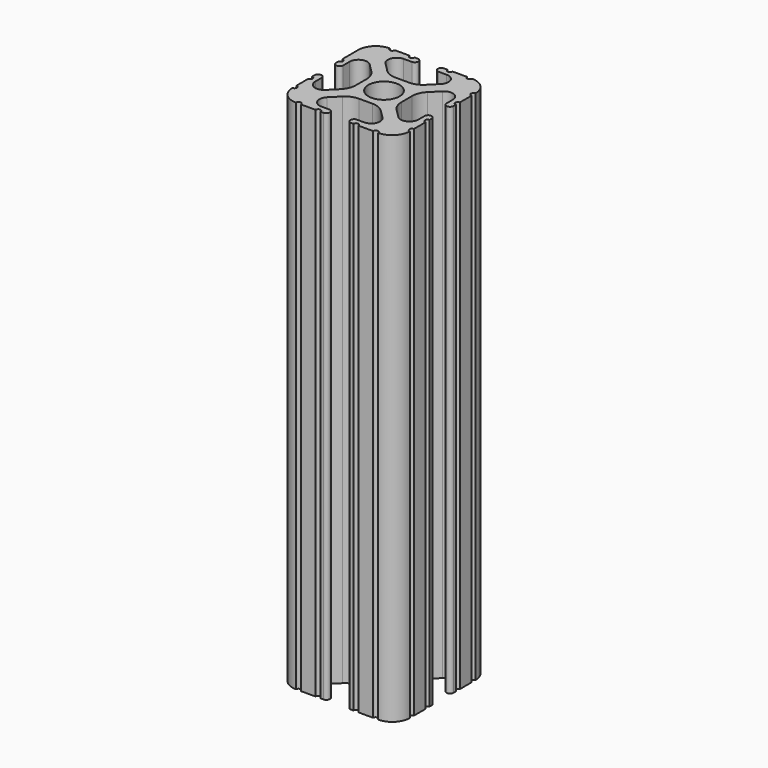
from build123d import *

# Parameters (mm, degrees)
F0_R     = 3.3625011168
F1_DEPTH = 111.76


# Not quite as in the source:
# - ends of sketch curves that miss each other by under 0.0002 mm in the source are joined


with BuildPart() as f1:
    # F0 (on Top) → F1 (new body)
    with BuildSketch(Plane.XY):
        with BuildLine():
            ThreePointArc((3.5659002011, 5.7489795053), (2.3298472421, 4.9230753228), (0.8718233648, 4.6330563417))
            Line((0.8718233648, 4.6330563417), (-2.0428700475, 4.6330563417))
            ThreePointArc((-2.0428700475, 4.6330563417), (-3.5008939248, 4.9230753228), (-4.7369468838, 5.7489795053))
            Line((-4.7369468838, 5.7489795053), (-6.5824285393, 7.5944611609))
            ThreePointArc((-6.5824285393, 7.5944611609), (-6.9953806306, 9.6705115177), (-5.2353901211, 10.846499579))
            Line((-5.2353901211, 10.846499579), (-3.5008939248, 10.846499579))
            Line((-3.5008939248, 10.846499579), (-3.4685428807, 10.846499579))
            ThreePointArc((-3.4685428807, 10.846499579), (-2.7109282724, 11.6201206221), (-3.4685428807, 12.3937416652))
            Line((-3.4685428807, 12.3937416652), (-3.5008939248, 12.3937416652))
            Line((-3.5008939248, 12.3937416652), (-4.1388643307, 12.3937416652))
            ThreePointArc((-4.1388643307, 12.3937416652), (-4.6871272259, 11.8525139305), (-5.2353901211, 12.3937416652))
            Line((-5.2353901211, 12.3937416652), (-8.3730050695, 12.3937416652))
            ThreePointArc((-8.3730050695, 12.3937416652), (-8.9242642054, 11.8424825293), (-9.4755233413, 12.3937416652))
            ThreePointArc((-9.4755233413, 12.3937416652), (-12.1696001777, 11.2778185015), (-13.2855233413, 8.5837416652))
            Line((-13.2855233413, 8.5837416652), (-13.2855233413, 7.4984658996))
            Line((-13.2855233413, 7.4984658996), (-13.2855233413, 4.343608445))
            ThreePointArc((-13.2855233413, 4.343608445), (-12.7296839168, 3.7964165708), (-13.2855233413, 3.2492246965))
            Line((-13.2855233413, 3.2492246965), (-13.2855233413, 2.6091122487))
            ThreePointArc((-13.2855233413, 2.6091122487), (-12.5119022982, 1.8532957784), (-11.7382812551, 2.6091122487))
            Line((-11.7382812551, 2.6091122487), (-11.7382812551, 4.343608445))
            ThreePointArc((-11.7382812551, 4.343608445), (-10.5622931938, 6.1035989545), (-8.486242837, 5.6906468632))
            Line((-8.486242837, 5.6906468632), (-6.6407611815, 3.8451652077))
            ThreePointArc((-6.6407611815, 3.8451652077), (-5.8148569989, 2.6091122487), (-5.5248380178, 1.1510883714))
            Line((-5.5248380178, 1.1510883714), (-5.5248380178, -1.7636050409))
            ThreePointArc((-5.5248380178, -1.7636050409), (-5.8148569989, -3.2216289182), (-6.6407611815, -4.4576818772))
            Line((-6.6407611815, -4.4576818772), (-8.486242837, -6.3031635328))
            ThreePointArc((-8.486242837, -6.3031635328), (-10.5622931938, -6.716115624), (-11.7382812551, -4.9561251146))
            Line((-11.7382812551, -4.9561251146), (-11.7382812551, -3.2216289182))
            ThreePointArc((-11.7382812551, -3.2216289182), (-12.5119022982, -2.4480078751), (-13.2855233413, -3.2216289182))
            Line((-13.2855233413, -3.2216289182), (-13.2855233413, -3.8570189362))
            Line((-13.2855233413, -3.8570189362), (-13.2855233413, -3.8595993241))
            ThreePointArc((-13.2855233413, -3.8595993241), (-12.7442956066, -4.4078622194), (-13.2855233413, -4.9561251146))
            Line((-13.2855233413, -4.9561251146), (-13.2855233413, -8.093740063))
            ThreePointArc((-13.2855233413, -8.093740063), (-12.9963771793, -8.175658031), (-12.7931661592, -8.3970656592))
            ThreePointArc((-12.7931661592, -8.3970656592), (-12.8130701183, -8.9360625991), (-13.2855233413, -9.1962583348))
            ThreePointArc((-13.2855233413, -9.1962583348), (-12.1696001777, -11.8903351711), (-9.4755233413, -13.0062583348))
            ThreePointArc((-9.4755233413, -13.0062583348), (-8.9263401234, -12.4513735034), (-8.3771569056, -13.0062583348))
            Line((-8.3771569056, -13.0062583348), (-5.2353901211, -13.0062583348))
            ThreePointArc((-5.2353901211, -13.0062583348), (-4.6881982469, -12.4504189103), (-4.1410063726, -13.0062583348))
            Line((-4.1410063726, -13.0062583348), (-3.5008939248, -13.0062583348))
            ThreePointArc((-3.5008939248, -13.0062583348), (-2.7450774545, -12.2326372917), (-3.5008939248, -11.4590162486))
            Line((-3.5008939248, -11.4590162486), (-5.2353901211, -11.4590162486))
            ThreePointArc((-5.2353901211, -11.4590162486), (-6.9953806306, -10.2830281872), (-6.5824285393, -8.2069778304))
            ThreePointArc((-6.5824285393, -8.2069778304), (-6.5813491493, -8.2058993046), (-6.5802706255, -8.2048199166))
            Line((-6.5802706255, -8.2048199166), (-4.7369468838, -6.3614961749))
            ThreePointArc((-4.7369468838, -6.3614961749), (-3.5008939248, -5.5355919924), (-2.0428700475, -5.2455730112))
            Line((-2.0428700475, -5.2455730112), (0.8718233648, -5.2455730112))
            ThreePointArc((0.8718233648, -5.2455730112), (2.3298472421, -5.5355919924), (3.5659002011, -6.3614961749))
            Line((3.5659002011, -6.3614961749), (5.4092239428, -8.2048199166))
            ThreePointArc((5.4092239428, -8.2048199166), (5.8221760341, -10.2808702734), (4.0621855247, -11.4568583348))
            Line((4.0621855247, -11.4568583348), (2.3298472421, -11.4568583348))
            ThreePointArc((2.3298472421, -11.4568583348), (1.7126411358, -12.2315583348), (2.3298472421, -13.0062583348))
            Line((2.3298472421, -13.0062583348), (2.9616088274, -13.0062583348))
            ThreePointArc((2.9616088274, -13.0062583348), (3.511897176, -12.460996221), (4.0621855247, -13.0062583348))
            Line((4.0621855247, -13.0062583348), (7.2156104858, -13.0062583348))
            ThreePointArc((7.2156104858, -13.0062583348), (7.7600435722, -12.4618252483), (8.3044766587, -13.0062583348))
            ThreePointArc((8.3044766587, -13.0062583348), (10.998553495, -11.8903351711), (12.1144766587, -9.1962583348))
            ThreePointArc((12.1144766587, -9.1962583348), (11.5750962663, -8.6501583348), (12.1144766587, -8.1040583348))
            Line((12.1144766587, -8.1040583348), (12.1144766587, -4.9539672008))
            ThreePointArc((12.1144766587, -4.9539672008), (11.570959409, -4.4045980675), (12.1144766587, -3.8552289343))
            Line((12.1144766587, -3.8552289343), (12.1144766587, -3.2216289182))
            ThreePointArc((12.1144766587, -3.2216289182), (11.3397766587, -2.5015675684), (10.5650766587, -3.2216289182))
            Line((10.5650766587, -3.2216289182), (10.5650766587, -4.9539672008))
            ThreePointArc((10.5650766587, -4.9539672008), (9.3890885973, -6.7139577102), (7.3130382405, -6.301005619))
            Line((7.3130382405, -6.301005619), (5.4697144988, -4.4576818772))
            ThreePointArc((5.4697144988, -4.4576818772), (4.6438103163, -3.2216289182), (4.3537913351, -1.7636050409))
            Line((4.3537913351, -1.7636050409), (4.3537913351, 1.1510883714))
            ThreePointArc((4.3537913351, 1.1510883714), (4.6438103163, 2.6091122487), (5.4697144988, 3.8451652077))
            Line((5.4697144988, 3.8451652077), (7.3130382405, 5.6884889494))
            ThreePointArc((7.3130382405, 5.6884889494), (9.3890885973, 6.1014410407), (10.5650766587, 4.3414505312))
            Line((10.5650766587, 4.3414505312), (10.5650766587, 2.6091122487))
            ThreePointArc((10.5650766587, 2.6091122487), (11.3397766587, 1.8731471479), (12.1144766587, 2.6091122487))
            Line((12.1144766587, 2.6091122487), (12.1144766587, 3.2492505312))
            ThreePointArc((12.1144766587, 3.2492505312), (11.5683766587, 3.7953505312), (12.1144766587, 4.3414505312))
            Line((12.1144766587, 4.3414505312), (12.1144766587, 7.4889068047))
            ThreePointArc((12.1144766587, 7.4889068047), (11.563421032, 8.0363242349), (12.1144766587, 8.5837416652))
            ThreePointArc((12.1144766587, 8.5837416652), (10.998553495, 11.2778185015), (8.3044766587, 12.3937416652))
            ThreePointArc((8.3044766587, 12.3937416652), (7.7491737928, 11.89736095), (7.1938709268, 12.3937416652))
            Line((7.1938709268, 12.3937416652), (4.0643434385, 12.3937416652))
            ThreePointArc((4.0643434385, 12.3937416652), (3.5181119113, 11.8531747523), (2.9718803841, 12.3937416652))
            Line((2.9718803841, 12.3937416652), (2.3298472421, 12.3937416652))
            Line((2.3298472421, 12.3937416652), (2.2582739116, 12.3937416652))
            ThreePointArc((2.2582739116, 12.3937416652), (1.5196122547, 11.6201206221), (2.2582739116, 10.846499579))
            Line((2.2582739116, 10.846499579), (2.3298472421, 10.846499579))
            Line((2.3298472421, 10.846499579), (4.0643434385, 10.846499579))
            ThreePointArc((4.0643434385, 10.846499579), (5.8243339479, 9.6705115177), (5.4113818566, 7.5944611609))
            Line((5.4113818566, 7.5944611609), (3.5659002011, 5.7489795053))
        make_face()
        with Locations((-0.5855233413, -0.3062583348)):
            Circle(F0_R, mode=Mode.SUBTRACT)
    extrude(amount=F1_DEPTH)


solid = f1.part
